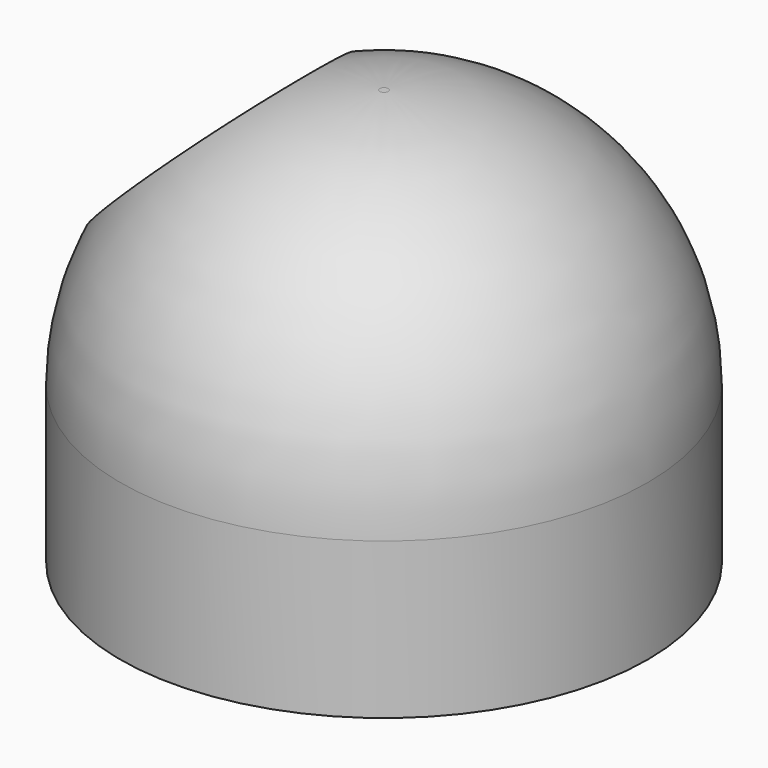
from build123d import *

# Parameters (mm, degrees)
F0_R     = 12.7
F1_DEPTH = 20
F2_R     = 12.5


# Not quite as in the source:
# - a fillet or chamfer that OpenCascade refuses, or shapes differently, is made with other operations: its cross-section is extruded or revolved along the edge and cut away or added


with BuildPart() as f1:
    # F0 (on Top) → F1 (new body)
    with BuildSketch(Plane.XY):
        Circle(F0_R)
    extrude(amount=F1_DEPTH)

    # F2
    f2_edges = [f1.edges().sort_by_distance(p)[0] for p in [
        (-12.7, 0, 20),
    ]]
    fillet(f2_edges, radius=F2_R)

    # F3 (on Front) → F4 (revolve, cut)
    with BuildSketch(Plane.XZ):
        Polygon((6.0710678119, 11.9289321881), (-1, 19), (-6.25, 13.75), (0.8210678119, 6.6789321881), align=None)
    revolve(axis=Axis((-2.7144660941, 0, 10.2144660941), (0.7071067812, 0, -0.7071067812)), mode=Mode.SUBTRACT)

    # F5 (on Front) → F6 (revolve, cut)
    with BuildSketch(Plane.XZ):
        with BuildLine():
            Line((-9.7855339059, 17.2855339059), (-5.1186291501, 12.6186291501))
            ThreePointArc((-5.1186291501, 12.6186291501), (-3.6879289914, 14.7598232523), (-3.1855339059, 17.2855339059))
            ThreePointArc((-3.1855339059, 17.2855339059), (-7.2598232523, 23.3831388205), (-14.4524386618, 21.9524386618))
            Line((-14.4524386618, 21.9524386618), (-9.7855339059, 17.2855339059))
        make_face()
    revolve(axis=Axis((-12.1189862838, 0, 19.6189862838), (-0.7071067812, 0, 0.7071067812)), mode=Mode.SUBTRACT)

    # F7: chamfer of 0.4 on 1 edges, made by hand

    # F7_s1 → F7_t2 (revolve, cut)
    with BuildSketch(Plane.XZ):
        with BuildLine():
            Line((-3.2011954465, 17.1809028584), (-2.9181547597, 17.0608682325))
            Line((-2.9181547597, 17.0608682325), (-2.9124979054, 17.0552113782))
            ThreePointArc((-2.9124979054, 17.0552113782), (-3.0605101564, 16.9281761351), (-3.1980339034, 16.7906523881))
            Line((-3.1980339034, 16.7906523881), (-3.2116687493, 16.7969022419))
            ThreePointArc((-3.2116687493, 16.7969022419), (-3.2002291645, 16.9885061916), (-3.2091943175, 17.1810372559))
            Line((-3.2091943175, 17.1810372559), (-3.2011954465, 17.1809028584))
        make_face()
    revolve(axis=Axis((-6.25, 0, 13.75), (-0.7071067812, 0, 0.7071067812)), mode=Mode.SUBTRACT)


solid = f1.part
